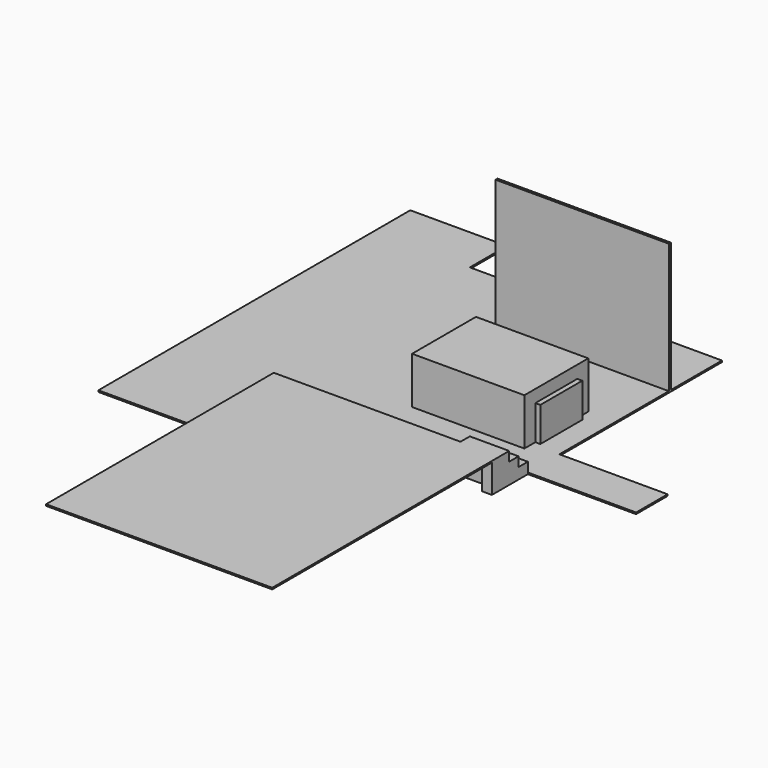
from build123d import *

# Parameters (mm, degrees)
F0_W      = 2250
F0_H      = 1600
F1_DEPTH  = 940
F0_W_2    = 500
F0_H_2    = 1800
F0_W_3    = 790
F0_H_3    = 700
F0_W_4    = 1800
F0_H_4    = 500
F2_DEPTH  = 30
F3_W      = 1050
F3_H      = 690
F4_DEPTH  = 100
F5_DEPTH  = 2600
F6_W      = 200
F6_H      = 200
F7_DEPTH  = 600
F9_DEPTH  = 30
F11_DEPTH = 790


# Not quite as in the source:
# - a feature names something its author has since deleted; it is built from what else it names


with BuildPart() as f1:
    # F0 (on Top) → F1 (new body)
    with BuildSketch(Plane.XY):
        Rectangle(F0_W, F0_H)
    extrude(amount=F1_DEPTH)

    # F0 (on Top) → F2 (join)
    with BuildSketch(Plane.XY):
        Polygon((1675, 2130), (3.0863761902, 2130), (-1796.9136238098, 2130), (-1796.9136238098, 2180), (1675, 2180), (1675, 3460), (-3375.1421768536, 3460), (-3375.1421768536, 4388.6961936951), (-5312.2445035196, 4388.6961936951), (-5312.2445035196, -3422.4522947772), (-2855.9122085571, -3422.4522947772), (-2855.9122085571, -2100), (-2855.9122085571, -300), (-2355.9122085571, -300), (-2355.9122085571, -2100), (-1255.9122085571, -2100), (-1255.9122085571, -1600), (544.0877914429, -1600), (544.0877914429, -2100), (885, -2100), (885, -1400), (1675, -1400), (1817.5126314163, -1400), (2516.7963504791, -1400), (3843.1406402588, -1400), (3843.1406402588, -610), (3053.1406402588, -610), (1675, -610), align=None)
        Rectangle(F0_W, F0_H, mode=Mode.SUBTRACT)
        with Locations((-2605.9122085571, -1200)):
            Rectangle(F0_W_2, F0_H_2)
        with Locations((1280, -1750)):
            Rectangle(F0_W_3, F0_H_3)
        Polygon((-1796.9136238098, 2130), (3.0863761902, 2130), (1675, 2130), (1675, 2180), (-1796.9136238098, 2180), align=None)
        Rectangle(F0_W, F0_H)
        with Locations((-355.9122085571, -1850)):
            Rectangle(F0_W_4, F0_H_4)
    extrude(amount=-F2_DEPTH)

    # F3 (on face) → F4 (join)
    with BuildSketch(Plane.YZ.offset(1125)):
        with Locations((0, 345)):
            Rectangle(F3_W, F3_H)
    extrude(amount=F4_DEPTH)

    # F0 (on Top) → F5 (join)
    with BuildSketch(Plane.XY):
        Polygon((-1796.9136238098, 2130), (3.0863761902, 2130), (1675, 2130), (1675, 2180), (-1796.9136238098, 2180), align=None)
    extrude(amount=F5_DEPTH)

    # F6 (on face) → F7 (join)
    with BuildSketch(Plane(origin=(0, 0, -30), x_dir=(1, 0, 0), z_dir=(0, 0, -1))):
        with Locations((-2755.9122085571, 2200)):
            Rectangle(F6_W, F6_H)
        with Locations((1575, 2200)):
            Rectangle(F6_W, F6_H)
    extrude(amount=-F7_DEPTH)

    # F8 (on face) → F9 (join)
    with BuildSketch(Plane.XY.offset(570)):
        Polygon((-2855.9122085571, -7802.6455282672), (1675, -7802.6455282672), (1675, -2100), (885, -2100), (544.0877914429, -2100), (-2855.9122085571, -2100), (-2855.9122085571, -3422.4522947772), align=None)
    extrude(amount=-F9_DEPTH)

    # F10 (on face) → F11 (join, through all)
    with BuildSketch(Plane.YZ.offset(1675)):
        Polygon((-1866.6666666667, 570), (-2100, 570), (-2100, 0), (-1400, 0), (-1400, 190), (-1633.3333333333, 190), (-1633.3333333333, 380), (-1866.6666666667, 380), align=None)
    extrude(amount=-F11_DEPTH)


solid = f1.part
